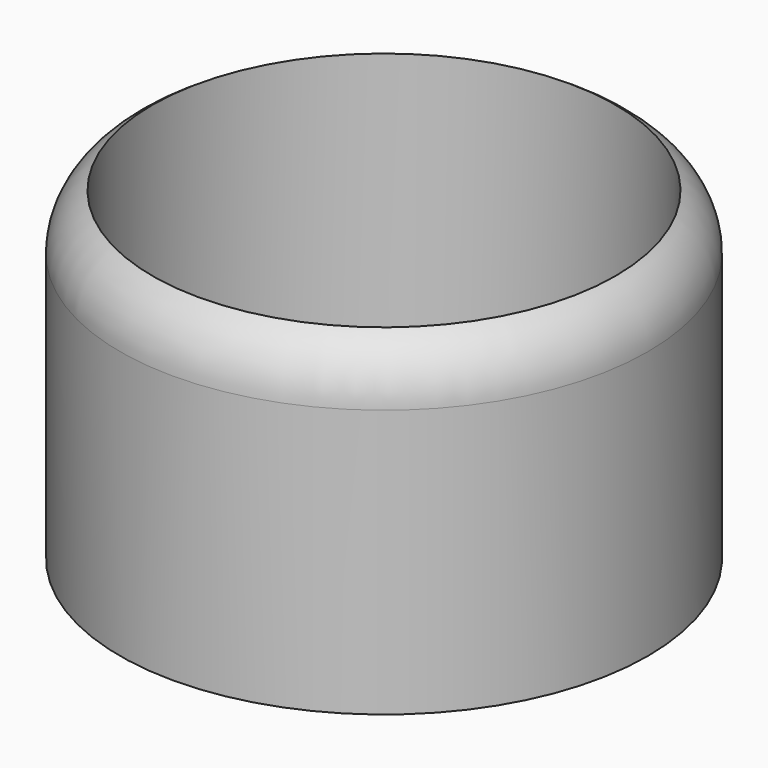
from build123d import *

# Parameters (mm, degrees)
F0_R     = 20.6945995874
F1_DEPTH = 25.4
F2_T     = -2.54


# Not quite as in the source:
# - a fillet or chamfer that OpenCascade refuses, or shapes differently, is made with other operations: its cross-section is extruded or revolved along the edge and cut away or added


with BuildPart() as f1:
    # F0 (on Top) → F1 (new body)
    with BuildSketch(Plane.XY):
        Circle(F0_R)
    extrude(amount=F1_DEPTH)

    # F2
    f2_openings = [f1.faces().sort_by_distance(p)[0] for p in [
        (0, 0, 25.4),
    ]]
    offset(amount=F2_T, openings=f2_openings)

    # F3: fillet of radius 5.08 on 1 edges, made by hand

    # F3_s1 → F3_t2 (revolve, cut)
    with BuildSketch(Plane.XZ):
        with BuildLine():
            ThreePointArc((20.6945995874, 21.0005909488), (20.0140086386, 23.5405909488), (18.1545995874, 25.4))
            Line((18.1545995874, 25.4), (20.6945995874, 25.4))
            Line((20.6945995874, 25.4), (20.6945995874, 21.0005909488))
        make_face()
    revolve(axis=Axis((0, 0, 25.4), (0, 0, 1)), mode=Mode.SUBTRACT)


solid = f1.part
